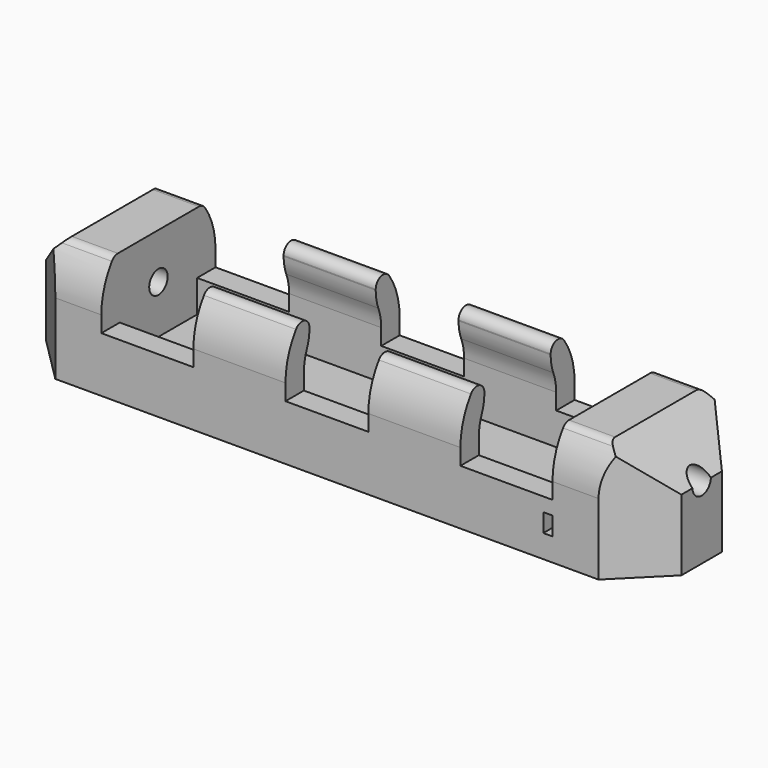
from build123d import *

# Parameters (mm, degrees)
F0_W         = 49
F0_H         = 15.5
F1_DEPTH     = 2.5
F3_DEPTH     = 49
F4_R         = 1
F5_R         = 5
F7_DEPTH     = 10
F9_DEPTH     = 10
F10_W        = 10
F10_H        = 6.7160013448
F10_W_2      = 9
F11_DEPTH    = 15.501
F12_T1_DEPTH = 36.7168298797
F12_T3_DEPTH = 33.4668298797
F13_R        = 1.25
F14_DEPTH    = 69.001
F15_W        = 1
F15_H        = 2
F16_DEPTH    = 15.501
F17_R        = 3.15
F18_DEPTH    = 1


# Not quite as in the source:
# - a fillet or chamfer that OpenCascade refuses, or shapes differently, is made with other operations: its cross-section is extruded or revolved along the edge and cut away or added


with BuildPart() as f1:
    # F0 (on Top) → F1 (new body)
    with BuildSketch(Plane.XY):
        with Locations((24.5, 7.75)):
            Rectangle(F0_W, F0_H)
    extrude(amount=F1_DEPTH)

    # F2 (on Right) → F3 (join, through all)
    with BuildSketch(Plane.YZ):
        with BuildLine():
            Line((0, 7.75), (0, 2.5))
            Line((0, 2.5), (2.5, 2.5))
            Line((2.5, 2.5), (2.5, 7.75))
            ThreePointArc((2.5, 7.75), (2.690862635, 9.1752192814), (3.25, 10.5))
            Line((3.25, 10.5), (3.25, 14.1449850143))
            ThreePointArc((3.25, 14.1449850143), (0.859115549, 11.3367232028), (0, 7.75))
        make_face()
        with BuildLine():
            Line((13, 7.75), (13, 2.5))
            Line((13, 2.5), (15.5, 2.5))
            Line((15.5, 2.5), (15.5, 7.75))
            ThreePointArc((15.5, 7.75), (14.640884451, 11.3367232028), (12.25, 14.1449850143))
            Line((12.25, 14.1449850143), (12.25, 10.5))
            ThreePointArc((12.25, 10.5), (12.809137365, 9.1752192814), (13, 7.75))
        make_face()
    extrude(amount=F3_DEPTH)

    # F4
    f4_edges = [f1.edges().sort_by_distance(p)[0] for p in [
        (24.5, 12.25, 14.144985),
        (24.5, 3.25, 14.144985),
    ]]
    fillet(f4_edges, radius=F4_R)

    # F5
    f5_edges = [f1.edges().sort_by_distance(p)[0] for p in [
        (24.5, 12.25, 10.5),
        (24.5, 3.25, 10.5),
    ]]
    fillet(f5_edges, radius=F5_R)

    # F6 (on face) → F7 (join)
    with BuildSketch(Plane(origin=(0, 0, 0), x_dir=(0, -1, 0), z_dir=(-1, 0, 0))):
        with BuildLine():
            ThreePointArc((-14.0692771084, 12.2893991295), (-15.1338520571, 10.1297642977), (-15.5, 7.75))
            Line((-15.5, 7.75), (-15.5, 0))
            Line((-15.5, 0), (0, 0))
            Line((0, 0), (0, 7.75))
            ThreePointArc((0, 7.75), (-0.3661479429, 10.1297642977), (-1.4307228916, 12.2893991295))
            ThreePointArc((-1.4307228916, 12.2893991295), (-1.7881546713, 12.6029618244), (-2.25, 12.7160013448))
            Line((-2.25, 12.7160013448), (-13.25, 12.7160013448))
            ThreePointArc((-13.25, 12.7160013448), (-13.7118453287, 12.6029618244), (-14.0692771084, 12.2893991295))
        make_face()
    extrude(amount=F7_DEPTH)

    # F8 (on face) → F9 (join)
    with BuildSketch(Plane.YZ.offset(49)):
        with BuildLine():
            Line((15.5, 0), (15.5, 7.75))
            ThreePointArc((15.5, 7.75), (15.1338520571, 10.1297642977), (14.0692771084, 12.2893991295))
            ThreePointArc((14.0692771084, 12.2893991295), (13.7118453287, 12.6029618244), (13.25, 12.7160013448))
            Line((13.25, 12.7160013448), (2.25, 12.7160013448))
            ThreePointArc((2.25, 12.7160013448), (1.7881546713, 12.6029618244), (1.4307228916, 12.2893991295))
            ThreePointArc((1.4307228916, 12.2893991295), (0.3661479429, 10.1297642977), (0, 7.75))
            Line((0, 7.75), (0, 0))
            Line((0, 0), (15.5, 0))
        make_face()
    extrude(amount=F9_DEPTH)

    # F10 (on face) → F11 (cut, through all)
    with BuildSketch(Plane.XZ):
        with Locations((44, 9.3580006724)):
            Rectangle(F10_W, F10_H)
        with Locations((24.5, 9.3580006724)):
            Rectangle(F10_W_2, F10_H)
        with Locations((5, 9.3580006724)):
            Rectangle(F10_W, F10_H)
    extrude(amount=-F11_DEPTH, mode=Mode.SUBTRACT)

    # F12: chamfer of 5 on 6 edges, made by hand

    # F12_s2 → F12_t1 (cut)
    with BuildSketch(Plane.XZ.offset(-26.1084149398)):
        Polygon((-10, 7.7160013448), (-5, 12.7160013448), (-10, 12.7160013448), align=None)
        Polygon((54, 12.7160013448), (59, 7.7160013448), (59, 12.7160013448), align=None)
    extrude(amount=F12_T1_DEPTH, mode=Mode.SUBTRACT)

    # F12_s4 → F12_t3 (cut)
    with BuildSketch(Plane.XY.offset(-12.8584149398)):
        Polygon((-10, 5), (-5, 0), (-10, 0), align=None)
        Polygon((-5, 15.5), (-10, 10.5), (-10, 15.5), align=None)
        Polygon((54, 0), (59, 5), (59, 0), align=None)
        Polygon((54, 15.5), (59, 10.5), (59, 15.5), align=None)
    extrude(amount=F12_T3_DEPTH, mode=Mode.SUBTRACT)

    # F13 (on face) → F14 (cut, through all)
    with BuildSketch(Plane(origin=(-10, 0, 0), x_dir=(0, -1, 0), z_dir=(-1, 0, 0))):
        with Locations((-7.75, 7.75)):
            Circle(F13_R)
    extrude(amount=-F14_DEPTH, mode=Mode.SUBTRACT)

    # F15 (on face) → F16 (cut, through all)
    with BuildSketch(Plane.XZ):
        with Locations((48.5, 3.5)):
            Rectangle(F15_W, F15_H)
    extrude(amount=-F16_DEPTH, mode=Mode.SUBTRACT)

    # F17 (on face) → F18 (cut)
    with BuildSketch(Plane(origin=(49, 0, 0), x_dir=(0, -1, 0), z_dir=(-1, 0, 0))):
        with Locations((-7.75, 7.75)):
            Circle(F17_R)
    extrude(amount=-F18_DEPTH, mode=Mode.SUBTRACT)


solid = f1.part
